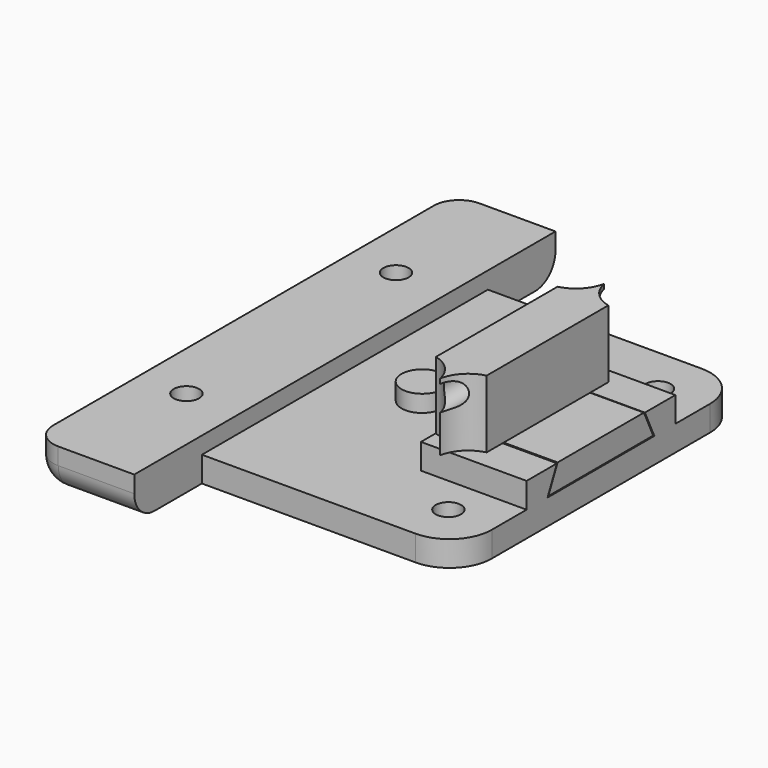
from build123d import *

# Parameters (mm, degrees)
F1_R          = 1.5
F1_R_2        = 2.45
F2_DEPTH      = 3
F3_W          = 12
F3_H          = 42.3
F3_R          = 3.3
F3_R_2        = 1.5
F4_DEPTH      = 2
F1_W          = 12
F1_H          = 10
F5_DEPTH      = 2
F6_R          = 3
F3_R_3        = 2.45
F7_DEPTH      = 2
F7_DEPTH_BACK = 3
F8_DEPTH      = 3
F9_T1_DEPTH   = 56.3
F9_T3_DEPTH   = 16.5
F9_T6_ANGLE   = 90
F9_T8_ANGLE   = 90
F10_W         = 12.5
F10_H         = 22
F11_DEPTH     = 3
F13_DEPTH     = 13
F15_DEPTH     = 12.5
F16_W         = 6
F16_H         = 12.7620736001
F17_DEPTH     = 8
F19_D         = 3
F19_DEPTH     = 42.3
F19_START     = 11.4989038
F19_TIP       = 0.9012909285


# Not quite as in the source:
# - a fillet or chamfer that OpenCascade refuses, or shapes differently, is made with other operations: its cross-section is extruded or revolved along the edge and cut away or added
# - a feature names something its author has since deleted; it is built from what else it names


with BuildPart() as f2:
    # F1 (on Top) → F2 (new body)
    with BuildSketch(Plane.XY):
        with BuildLine():
            Line((-7.9588235294, 20.0470588235), (-19.9588235294, 20.0470588235))
            Line((-19.9588235294, 20.0470588235), (-19.9588235294, -22.2529411765))
            Line((-19.9588235294, -22.2529411765), (-7.9588235294, -22.2529411765))
            Line((-7.9588235294, -22.2529411765), (17.3411764706, -22.2529411765))
            ThreePointArc((17.3411764706, -22.2529411765), (20.8767103765, -20.7884750824), (22.3411764706, -17.2529411765))
            Line((22.3411764706, -17.2529411765), (22.3411764706, 15.0470588235))
            ThreePointArc((22.3411764706, 15.0470588235), (20.8767103765, 18.5825927295), (17.3411764706, 20.0470588235))
            Line((17.3411764706, 20.0470588235), (-7.9588235294, 20.0470588235))
        make_face()
        with Locations((-14.3088235294, -16.6029411765)):
            Circle(F1_R, mode=Mode.SUBTRACT)
        with Locations((1.1911764706, -1.1029411765)):
            Circle(F1_R_2, mode=Mode.SUBTRACT)
        with Locations((16.6911764706, -16.6029411765)):
            Circle(F1_R, mode=Mode.SUBTRACT)
        with Locations((-14.3088235294, 14.3970588235)):
            Circle(F1_R, mode=Mode.SUBTRACT)
        with Locations((16.6911764706, 14.3970588235)):
            Circle(F1_R, mode=Mode.SUBTRACT)
    extrude(amount=F2_DEPTH)

    # F3 (on face) → F4 (join)
    with BuildSketch(Plane.XY.offset(3)):
        with Locations((-13.9588235294, -1.1029411765)):
            Rectangle(F3_W, F3_H)
        with Locations((-14.3088235294, -16.6029411765)):
            Circle(F3_R, mode=Mode.SUBTRACT)
        with Locations((-14.3088235294, 14.3970588235)):
            Circle(F3_R, mode=Mode.SUBTRACT)
        with Locations((-14.3088235294, 14.3970588235)):
            Circle(F3_R)
        with Locations((-14.3088235294, 14.3970588235)):
            Circle(F3_R_2, mode=Mode.SUBTRACT)
        with Locations((-14.3088235294, -16.6029411765)):
            Circle(F3_R)
        with Locations((-14.3088235294, -16.6029411765)):
            Circle(F3_R_2, mode=Mode.SUBTRACT)
    extrude(amount=F4_DEPTH)

    # F1 (on Top) → F5 (join)
    with BuildSketch(Plane.XY):
        with Locations((-13.9588235294, 25.0470588235)):
            Rectangle(F1_W, F1_H)
        with Locations((-13.9588235294, -27.2529411765)):
            Rectangle(F1_W, F1_H)
    extrude(amount=F5_DEPTH)

    # F6
    f6_edges = [f2.edges().sort_by_distance(p)[0] for p in [
        (-19.958824, -32.252941, 1),
        (-19.958824, 30.047059, 1),
    ]]
    fillet(f6_edges, radius=F6_R)

    # F3 (on face) → F7 (join, two sides)
    with BuildSketch(Plane.XY.offset(3)) as f7_sk:
        with Locations((1.1911764706, -1.1029411765)):
            Circle(F3_R_3)
    extrude(amount=F7_DEPTH)
    extrude(f7_sk.sketch, amount=-F7_DEPTH_BACK)

    # F8 (add): faces of the model
    f8_faces = [f2.faces().sort_by_distance(p)[0] for p in [
        (-13.8716348016, 24.9762285246, 2),
        (-13.8716348016, -27.1821108776, 2),
    ]]
    extrude(f8_faces, amount=F8_DEPTH)

    # F9: fillet of radius 3 on 5 edges, made by hand

    # F9_s2 → F9_t1 (cut)
    with BuildSketch(Plane.XZ.offset(-27.0470588235)):
        with BuildLine():
            ThreePointArc((-19.9588235294, 3), (-19.080143873, 0.8786796564), (-16.9588235294, 0))
            Line((-16.9588235294, 0), (-19.9588235294, 0))
            Line((-19.9588235294, 0), (-19.9588235294, 3))
        make_face()
    extrude(amount=F9_T1_DEPTH, mode=Mode.SUBTRACT)

    # F9_s4 → F9_t3 (cut)
    with BuildSketch(Plane.YZ.offset(-16.9588235294)):
        with BuildLine():
            ThreePointArc((30.0470588235, 3), (29.1683791671, 0.8786796564), (27.0470588235, 0))
            Line((27.0470588235, 0), (30.0470588235, 0))
            Line((30.0470588235, 0), (30.0470588235, 3))
        make_face()
        with BuildLine():
            ThreePointArc((-32.2529411765, 3), (-31.37426152, 0.8786796564), (-29.2529411765, 0))
            Line((-29.2529411765, 0), (-32.2529411765, 0))
            Line((-32.2529411765, 0), (-32.2529411765, 3))
        make_face()
    extrude(amount=F9_T3_DEPTH, mode=Mode.SUBTRACT)

    # F9_s5 → F9_t6 (revolve, cut)
    with BuildSketch(Plane.XZ.offset(-27.0470588235)):
        with BuildLine():
            ThreePointArc((-19.9588235294, 3), (-19.080143873, 0.8786796564), (-16.9588235294, 0))
            Line((-16.9588235294, 0), (-19.9588235294, 0))
            Line((-19.9588235294, 0), (-19.9588235294, 3))
        make_face()
    revolve(axis=Axis((-16.9588235294, 27.0470588235, 0), (0, 0, -1)), revolution_arc=F9_T6_ANGLE, mode=Mode.SUBTRACT)

    # F9_s7 → F9_t8 (revolve, cut)
    with BuildSketch(Plane.XZ.offset(29.2529411765)):
        with BuildLine():
            ThreePointArc((-16.9588235294, 0), (-19.080143873, 0.8786796564), (-19.9588235294, 3))
            Line((-19.9588235294, 3), (-19.9588235294, 0))
            Line((-19.9588235294, 0), (-16.9588235294, 0))
        make_face()
    revolve(axis=Axis((-16.9588235294, -29.2529411765, 0), (0, 0, 1)), revolution_arc=F9_T8_ANGLE, mode=Mode.SUBTRACT)

    # F10 (on face) → F11 (join)
    with BuildSketch(Plane.XY.offset(3)):
        with Locations((16.0911764706, -1.1029411765)):
            Rectangle(F10_W, F10_H)
    extrude(amount=F11_DEPTH)

    # F12 (on face) → F13 (cut)
    with BuildSketch(Plane.YZ.offset(22.3411764706)):
        Polygon((5.3970588235, 6), (-7.6029411765, 6), (-9.0018641509, 3), (6.795981798, 3), align=None)
    extrude(amount=-F13_DEPTH, mode=Mode.SUBTRACT)


with BuildPart() as f15:
    # F14 (on face) → F15 (new body)
    with BuildSketch(Plane.YZ.offset(22.3411764706)):
        Polygon((6.6231914472, 3.1115159904), (5.2496820965, 6.0570162982), (-7.5123915035, 6.0570162982), (-8.8859008542, 3.1115159904), align=None)
    extrude(amount=-F15_DEPTH)

    # F16 (on face) → F17 (join)
    with BuildSketch(Plane.XY.offset(6.0570162982)):
        with BuildLine():
            ThreePointArc((12.9661764706, 11.1031076104), (11.9330087808, 9.0817074362), (9.9661764706, 7.9481004483))
            Line((9.9661764706, 7.9481004483), (9.9661764706, 5.2496820965))
            Line((9.9661764706, 5.2496820965), (15.9661764706, 5.2496820965))
            Line((15.9661764706, 5.2496820965), (15.9661764706, 7.9481004483))
            ThreePointArc((15.9661764706, 7.9481004483), (13.9993441603, 9.0817074362), (12.9661764706, 11.1031076104))
        make_face()
        with Locations((12.9661764706, -1.1313547035)):
            Rectangle(F16_W, F16_H)
        with BuildLine():
            Line((15.9661764706, -7.5123915035), (9.9661764706, -7.5123915035))
            Line((9.9661764706, -7.5123915035), (9.9661764706, -10.0418852275))
            ThreePointArc((9.9661764706, -10.0418852275), (11.9330087808, -11.1754922153), (12.9661764706, -13.1968923896))
            ThreePointArc((12.9661764706, -13.1968923896), (13.9993441603, -11.1754922153), (15.9661764706, -10.0418852275))
            Line((15.9661764706, -10.0418852275), (15.9661764706, -7.5123915035))
        make_face()
    extrude(amount=F17_DEPTH)

    # F19
    # its depths count from where the whole tool has entered the part; down to there all is cleared
    with Locations(Plane.XZ.offset(22.2529411765).offset(-F19_START)):
        with Locations((12.9636181518, 12)):
            Hole(F19_D / 2, depth=F19_DEPTH)
            with Locations((0, 0, -(F19_DEPTH + F19_TIP / 2))):  # 118° drill point
                Cone(0, F19_D / 2, F19_TIP, mode=Mode.SUBTRACT)


solid = Compound([f2.part, f15.part])
